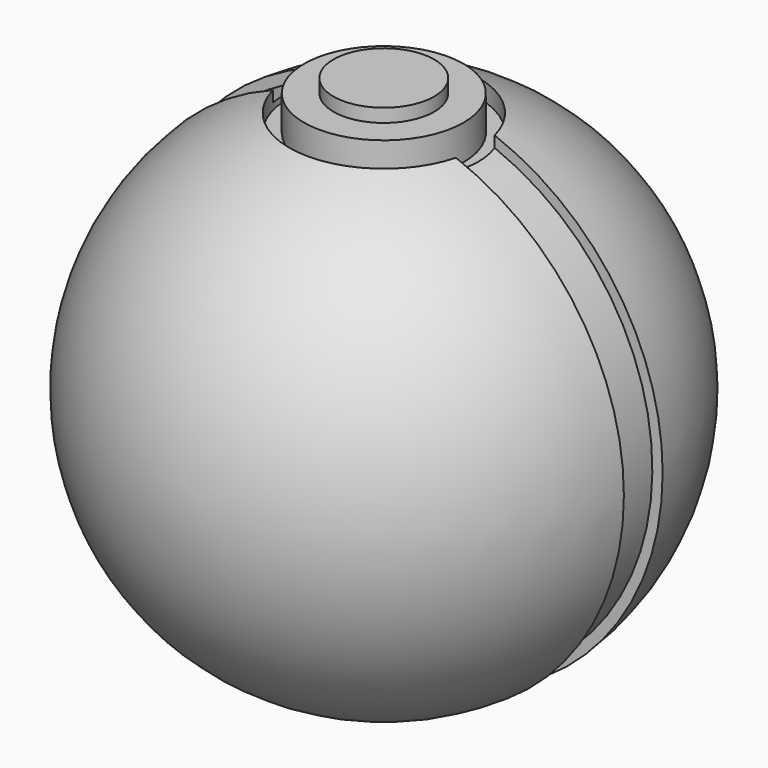
from build123d import *

# Parameters (mm, degrees)
F3_R     = 4.7700695271
F4_DEPTH = 25.908
F5_R     = 7.5557207763
F6_DEPTH = 24.638
F7_R     = 8.9716016728
F7_R_2   = 7.5557207763
F8_DEPTH = 3.302


# Not quite as in the source:
# - a feature names something its author has since deleted; it is built from what else it names


with BuildPart() as f2:
    # F0 (on Top) → F2 (revolve)
    with BuildSketch(Plane.XY):
        with BuildLine():
            Line((0, 24.6944446117), (0, -24.6944446117))
            ThreePointArc((0, -24.6944446117), (16.6301779866, -18.2552122643), (24.5875081551, -2.2956562028))
            Line((24.5875081551, -2.2956562028), (23.6113984138, -2.2956562028))
            Line((23.6113984138, -2.2956562028), (23.6113984138, 2.2956562028))
            Line((23.6113984138, 2.2956562028), (24.5875081551, 2.2956562028))
            ThreePointArc((24.5875081551, 2.2956562028), (16.6301779866, 18.2552122643), (0, 24.6944446117))
        make_face()
    revolve(axis=Axis((0, 0.329259783, 0), (0, -1, 0)))

    # F3 (on Top) → F4 (join)
    with BuildSketch(Plane.XY):
        Circle(F3_R)
    extrude(amount=F4_DEPTH)

    # F5 (on Top) → F6 (join)
    with BuildSketch(Plane.XY):
        Circle(F5_R)
    extrude(amount=F6_DEPTH)

    # F7 (on face) → F8 (cut)
    with BuildSketch(Plane.XY.offset(24.638)):
        Circle(F7_R)
        Circle(F7_R_2, mode=Mode.SUBTRACT)
    extrude(amount=-F8_DEPTH, mode=Mode.SUBTRACT)


solid = f2.part
